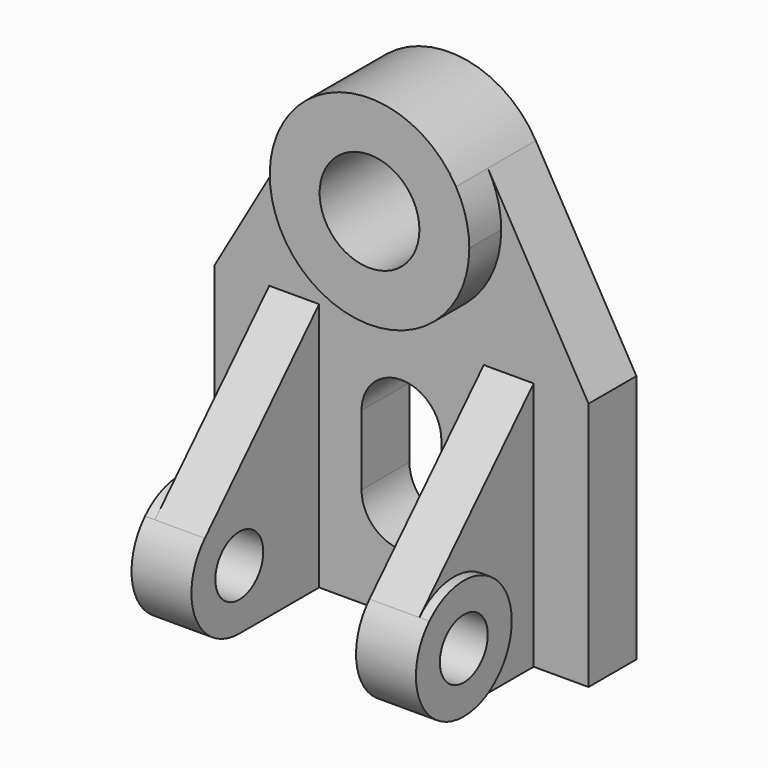
from build123d import *

# Parameters (mm, degrees)
F1_DEPTH = 12
F0_R     = 10
F2_DEPTH = 20
F5_DEPTH = 10
F4_R     = 6
F6_DEPTH = 12


# Not quite as in the source:
# - a pattern or mirror of a feature is missing from the dataset's text; its kind, count and spacing are read off the source's solid


with BuildPart() as f1:
    # F0 (on Front) → F1 (new body)
    with BuildSketch(Plane.XZ):
        with BuildLine():
            ThreePointArc((17.3264581055, 84.9896871582), (19.3200564454, 80.1706304205), (20, 75))
            ThreePointArc((20, 75), (-5.1706304205, 55.6799435546), (-17.3264581055, 84.9896871582))
            Line((-17.3264581055, 84.9896871582), (-37.5, 50))
            Line((-37.5, 50), (-37.5, 0))
            Line((-37.5, 0), (37.5, 0))
            Line((37.5, 0), (37.5, 50))
            Line((37.5, 50), (17.3264581055, 84.9896871582))
        make_face()
        with BuildLine():
            ThreePointArc((8, 20), (0, 12), (-8, 20))
            Line((-8, 20), (-8, 34))
            ThreePointArc((-8, 34), (0, 42), (8, 34))
            Line((8, 34), (8, 20))
        make_face(mode=Mode.SUBTRACT)
    extrude(amount=F1_DEPTH)

    # F0 (on Front) → F2 (join)
    with BuildSketch(Plane.XZ):
        with BuildLine():
            ThreePointArc((-17.3264581055, 84.9896871582), (-5.1706304205, 55.6799435546), (20, 75))
            ThreePointArc((20, 75), (19.3200564454, 80.1706304205), (17.3264581055, 84.9896871582))
            ThreePointArc((17.3264581055, 84.9896871582), (0, 95), (-17.3264581055, 84.9896871582))
        make_face()
        with Locations((0, 75)):
            Circle(F0_R, mode=Mode.SUBTRACT)
    extrude(amount=F2_DEPTH)

    # F4 (on offset) → F5 (join)
    with BuildSketch(Plane.YZ.offset(16.5)):
        with BuildLine():
            ThreePointArc((-40.6341440633, 20.3337600333), (-27.5061001769, 23.1267634279), (-20, 12))
            ThreePointArc((-20, 12), (-23.5147186258, 3.5147186258), (-32, 0))
            Line((-32, 0), (-12, 0))
            Line((-12, 0), (-12, 50))
            Line((-12, 50), (-40.6341440633, 20.3337600333))
        make_face()
    f5 = extrude(amount=F5_DEPTH)

    # F5_copies: F5 across plane
    add(f5.mirror(Plane(origin=(0, 0, 0), x_dir=(0, 0, -1), z_dir=(-1, 0, 0))))

    # F4 (on offset) → F6 (join)
    with BuildSketch(Plane.YZ.offset(16.5)):
        with BuildLine():
            ThreePointArc((-32, 0), (-23.5147186258, 3.5147186258), (-20, 12))
            ThreePointArc((-20, 12), (-27.5061001769, 23.1267634279), (-40.6341440633, 20.3337600333))
            ThreePointArc((-40.6341440633, 20.3337600333), (-43.0454769114, 7.3098571664), (-32, 0))
        make_face()
        with Locations((-32, 12)):
            Circle(F4_R, mode=Mode.SUBTRACT)
    f6 = extrude(amount=F6_DEPTH)

    # F6_copies: F6 across plane
    add(f6.mirror(Plane(origin=(0, 0, 0), x_dir=(0, 0, -1), z_dir=(-1, 0, 0))))


solid = f1.part
